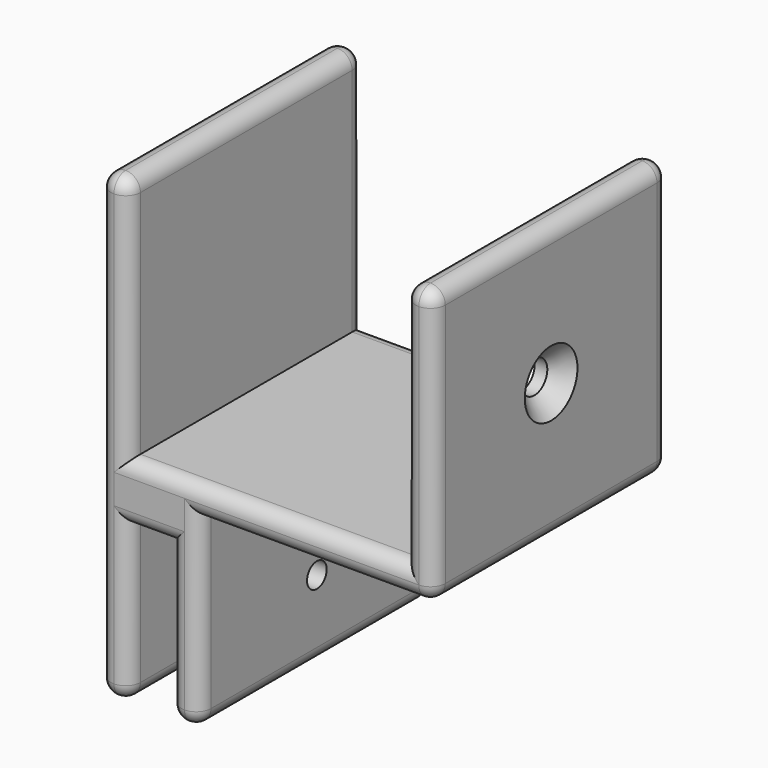
from build123d import *

# Parameters (mm, degrees)
F1_DEPTH       = 30
F3_D           = 3.3
F3_DEPTH       = 13.5
F3_CSINK_D     = 6.72
F3_CSINK_ANGLE = 90
F3_TIP         = 0.9914200214
F4_R           = 1.49999
F6_D           = 3.3
F6_DEPTH       = 7
F6_CSINK_D     = 6.72
F6_CSINK_ANGLE = 90
F6_TIP         = 0.9914200214
F8_D           = 2.5
F8_DEPTH       = 7
F8_TIP         = 0.7510757738


# Not quite as in the source:
# - a fillet or chamfer is up to 0.001 mm smaller than in the source, because OpenCascade refuses the exact size


with BuildPart() as f1:
    # F0 (on Front) → F1 (new body)
    with BuildSketch(Plane.XZ):
        Polygon((0, 28), (0, 0), (0, -19), (3, -19), (3, -3), (7.2, -3), (7.2, -19), (10.2, -19), (10.2, 0), (34.1, 0), (34.1, 28), (31.1, 28), (31.1, 3), (3, 3), (3, 28), align=None)
    extrude(amount=F1_DEPTH)

    # F3
    with Locations(Plane.YZ.offset(34.1)):
        with Locations((-15, 14)):
            CounterSinkHole(F3_D / 2, F3_CSINK_D / 2, depth=F3_DEPTH, counter_sink_angle=F3_CSINK_ANGLE)
            with Locations((0, 0, -(F3_DEPTH + F3_TIP / 2))):  # 118° drill point
                Cone(0, F3_D / 2, F3_TIP, mode=Mode.SUBTRACT)

    # F4 (radius 1.5 in the source; OpenCascade refuses exactly that, so slightly less here)
    f4_edges = [f1.edges().sort_by_distance(p)[0] for p in [
        (0, -15, -19),
        (3, -15, -19),
        (7.2, -15, -19),
        (10.2, -15, -19),
        (31.1, -15, 28),
        (34.1, -15, 28),
        (3, -15, 28),
        (0, -15, 28),
        (1.5, -30, 28),
        (32.6, -30, 28),
        (31.1, -30, 15.5),
        (34.1, -30, 14),
        (3, -30, 15.5),
        (0, -30, 4.5),
        (17.05, -30, 3),
        (22.15, -30, 0),
        (10.2, -30, -9.5),
        (1.5, -30, -19),
        (8.7, -30, -19),
        (1.5, 0, -19),
        (8.7, 0, -19),
        (0, 0, 4.5),
        (3, 0, -11),
        (7.2, 0, -11),
        (10.2, 0, -9.5),
        (17.05, 0, 3),
        (3, 0, 15.5),
        (22.15, 0, 0),
        (34.1, 0, 14),
        (34.1, -15, 0),
        (5.1, 0, -3),
        (5.1, -30, -3),
        (32.6, 0, 28),
        (1.5, 0, 28),
        (31.1, 0, 15.5),
        (3, -30, -11),
        (7.2, -30, -11),
    ]]
    fillet(f4_edges, radius=F4_R)

    # F6
    with Locations(Plane(origin=(0, 0, 0), x_dir=(0, -1, 0), z_dir=(-1, 0, 0))):
        with Locations((15, -11)):
            CounterSinkHole(F6_D / 2, F6_CSINK_D / 2, depth=F6_DEPTH, counter_sink_angle=F6_CSINK_ANGLE)
            with Locations((0, 0, -(F6_DEPTH + F6_TIP / 2))):  # 118° drill point
                Cone(0, F6_D / 2, F6_TIP, mode=Mode.SUBTRACT)

    # F8
    with Locations(Plane.YZ.offset(10.2)):
        with Locations((-15, -11)):
            Hole(F8_D / 2, depth=F8_DEPTH)
            with Locations((0, 0, -(F8_DEPTH + F8_TIP / 2))):  # 118° drill point
                Cone(0, F8_D / 2, F8_TIP, mode=Mode.SUBTRACT)


solid = f1.part
